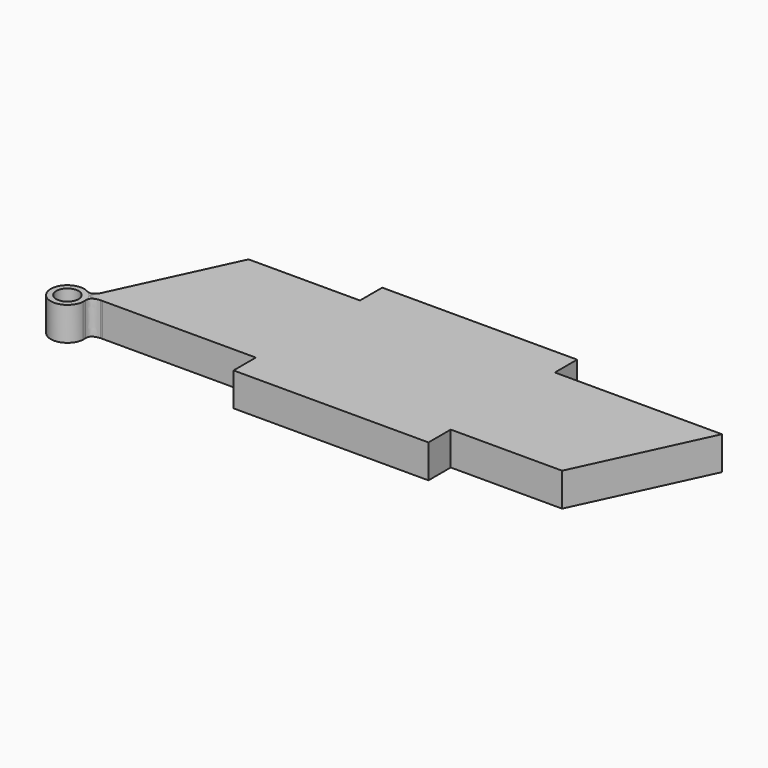
from build123d import *

# Parameters (mm, degrees)
F1_DEPTH = 6
F0_R     = 2
F2_DEPTH = 6


with BuildPart() as f1:
    # F0 (on Top) → F1 (new body)
    with BuildSketch(Plane.XY):
        with BuildLine():
            Line((-50.0249465513, 29.52996234), (-50.5862181266, 28.3271253868))
            Line((-50.5862181266, 28.3271253868), (-48.5040023923, 28.3271253868))
            add(Edge.make_bspline(
                [(-48.5040023923, 28.3271253868), (-48.3265830997, 28.3410976173), (-48.2191282446, 28.3290178572), (-48.177883029, 28.3271253868)],
                knots=[0.7675517488, 0.7675517488, 0.7675517488, 0.7675517488, 0.9509774258, 0.9509774258, 0.9509774258, 0.9509774258], degree=3))
            Line((-48.177883029, 28.3271253868), (-48.1545887887, 28.3271253868))
            Line((-48.1545887887, 28.3271253868), (-20.5862181266, 28.3271253868))
            Line((-20.5862181266, 28.3271253868), (-20.5862181266, 23.3271253868))
            Line((-20.5862181266, 23.3271253868), (14.4137818734, 23.3271253868))
            Line((14.4137818734, 23.3271253868), (14.4137818734, 28.3271253868))
            Line((14.4137818734, 28.3271253868), (34.4137818734, 28.3271253868))
            Line((34.4137818734, 28.3271253868), (44.9851090482, 50.9820816164))
            Line((44.9851090482, 50.9820816164), (14.9851090482, 50.9820816164))
            Line((14.9851090482, 50.9820816164), (14.9851090482, 55.9820816164))
            Line((14.9851090482, 55.9820816164), (-20.0148909518, 55.9820816164))
            Line((-20.0148909518, 55.9820816164), (-20.0148909518, 50.9820816164))
            Line((-20.0148909518, 50.9820816164), (-40.0148909518, 50.9820816164))
            Line((-40.0148909518, 50.9820816164), (-49.8350928217, 29.9368296959))
            add(Edge.make_bspline(
                [(-49.8350928217, 29.9368296959), (-49.8287783598, 29.9415238557), (-49.8442396119, 29.9138038591), (-49.8624208334, 29.8782642102)],
                knots=[0.6997217006, 0.6997217006, 0.6997217006, 0.6997217006, 0.7870450964, 0.7870450964, 0.7870450964, 0.7870450964], degree=3))
            Line((-49.8624208334, 29.8782642102), (-50.0249465513, 29.52996234))
        make_face()
    extrude(amount=F1_DEPTH)

    # F0 (on Top) → F2, piece 3 (join)
    with BuildSketch(Plane.XY):
        with BuildLine():
            Line((-48.1545887887, 28.3271253868), (-48.177883029, 28.3271253868))
            add(Edge.make_bspline(
                [(-48.177883029, 28.3271253868), (-48.1668597814, 28.3266196028), (-48.1605657938, 28.3268414823), (-48.1545887887, 28.3271253868)],
                knots=[0.9509774258, 0.9509774258, 0.9509774258, 0.9509774258, 1, 1, 1, 1], degree=3))
        make_face()
    extrude(amount=F2_DEPTH)


with BuildPart() as f1b:
    # F0 (on Top) → F1, piece 2 (new body)
    with BuildSketch(Plane.XY):
        with BuildLine():
            ThreePointArc((-50.0990342752, 27.0268241237), (-50.2663592156, 27.7055497053), (-50.5862181266, 28.3271253868))
            ThreePointArc((-50.5862181266, 28.3271253868), (-51.0346189675, 28.851670583), (-51.5910155934, 29.2598785833))
            ThreePointArc((-51.5910155934, 29.2598785833), (-55.7260895801, 25.2475821047), (-50.0847692352, 26.4192751848))
            add(Edge.make_bspline(
                [(-50.0847692352, 26.4192751848), (-50.0886085443, 26.6089058035), (-50.1045665089, 26.8197544117), (-50.0990342752, 27.0268241237)],
                knots=[0, 0, 0, 0, 0.1607658778, 0.1607658778, 0.1607658778, 0.1607658778], degree=3))
        make_face()
        with Locations((-53.0756514359, 26.6529922385)):
            Circle(F0_R, mode=Mode.SUBTRACT)
    extrude(amount=F1_DEPTH)


with BuildPart() as f2:
    # F0 (on Top) → F2 (new body)
    with BuildSketch(Plane.XY):
        with BuildLine():
            ThreePointArc((-51.5910155934, 29.2598785833), (-51.0346189675, 28.851670583), (-50.5862181266, 28.3271253868))
            Line((-50.5862181266, 28.3271253868), (-50.0249465513, 29.52996234))
            add(Edge.make_bspline(
                [(-49.8624208334, 29.8782642102), (-49.9067592406, 29.7915939378), (-49.9672739064, 29.6584184674), (-50.0249465513, 29.52996234)],
                knots=[0.7870450964, 0.7870450964, 0.7870450964, 0.7870450964, 1, 1, 1, 1], degree=3))
            Line((-49.8624208334, 29.8782642102), (-49.8350928217, 29.9368296959))
            add(Edge.make_bspline(
                [(-51.5910155934, 29.2598785833), (-51.3183012558, 29.1677802311), (-50.6411432567, 28.7943490334), (-49.8614766476, 29.9172160064), (-49.8350928217, 29.9368296959)],
                knots=[0, 0, 0, 0, 0.3348568359, 0.6997217006, 0.6997217006, 0.6997217006, 0.6997217006], degree=3))
        make_face()
    extrude(amount=F2_DEPTH)


with BuildPart() as f2b:
    # F0 (on Top) → F2, piece 2 (new body)
    with BuildSketch(Plane.XY):
        with BuildLine():
            Line((-48.5040023923, 28.3271253868), (-50.5862181266, 28.3271253868))
            ThreePointArc((-50.5862181266, 28.3271253868), (-50.2663592156, 27.7055497053), (-50.0990342752, 27.0268241237))
            add(Edge.make_bspline(
                [(-50.0990342752, 27.0268241237), (-50.091596006, 27.3052361266), (-49.9616584893, 28.0676117598), (-48.8818418367, 28.2973695484), (-48.5040023923, 28.3271253868)],
                knots=[0.1607658778, 0.1607658778, 0.1607658778, 0.1607658778, 0.3769208605, 0.7675517488, 0.7675517488, 0.7675517488, 0.7675517488], degree=3))
        make_face()
    extrude(amount=F2_DEPTH)


solid = Compound([f1.part, f1b.part, f2.part, f2b.part])
